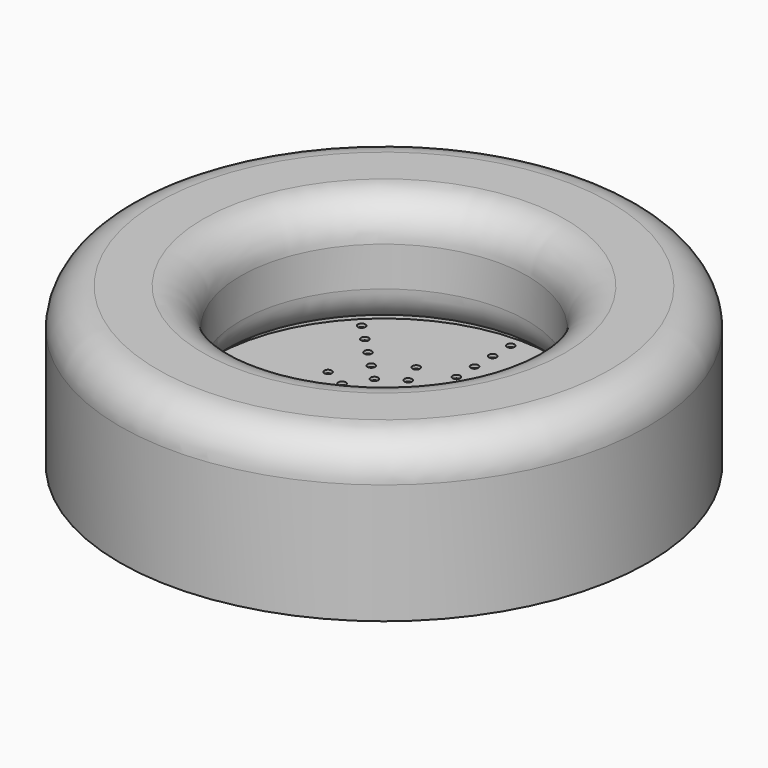
from build123d import *

# Parameters (mm, degrees)
F0_R      = 35
F0_R_2    = 20
F1_DEPTH  = 2
F2_R      = 35
F2_R_2    = 32
F3_DEPTH  = 3
F4_R      = 35
F5_DEPTH  = 0.4
F6_R      = 0.5
F7_DEPTH  = 1
F8_R      = 35
F8_R_2    = 22.5
F9_DEPTH  = 0.5
F10_R     = 35
F10_R_2   = 22.5
F10_R_3   = 19
F11_DEPTH = 15


# Not quite as in the source:
# - a fillet or chamfer that OpenCascade refuses, or shapes differently, is made with other operations: its cross-section is extruded or revolved along the edge and cut away or added


with BuildPart() as f1:
    # F0 (on Top) → F1 (new body)
    with BuildSketch(Plane.XY):
        Circle(F0_R)
        Circle(F0_R_2, mode=Mode.SUBTRACT)
    extrude(amount=F1_DEPTH)

    # F2 (on face) → F3 (join)
    with BuildSketch(Plane.XY.offset(2)):
        Circle(F2_R)
        Circle(F2_R_2, mode=Mode.SUBTRACT)
    extrude(amount=F3_DEPTH)

    # F4 (on face) → F5 (join)
    with BuildSketch(Plane.XY.offset(5)):
        Circle(F4_R)
    extrude(amount=F5_DEPTH)

    # F6 (on face) → F7 (cut)
    with BuildSketch(Plane.XY.offset(5.4)):
        Circle(F6_R)
        with Locations((3, 0)):
            Circle(F6_R)
        with Locations((6, 0)):
            Circle(F6_R)
        with Locations((9, 0)):
            Circle(F6_R)
        with Locations((12, 0)):
            Circle(F6_R)
        with Locations((15, 0)):
            Circle(F6_R)
        with Locations((18, 0)):
            Circle(F6_R)
        with Locations((21, 0)):
            Circle(F6_R)
        with Locations((2.1213203436, 2.1213203436)):
            Circle(F6_R)
        with Locations((4.2426406871, 4.2426406871)):
            Circle(F6_R)
        with Locations((6.3639610307, 6.3639610307)):
            Circle(F6_R)
        with Locations((8.4852813742, 8.4852813742)):
            Circle(F6_R)
        with Locations((10.6066017178, 10.6066017178)):
            Circle(F6_R)
        with Locations((12.7279220614, 12.7279220614)):
            Circle(F6_R)
        with Locations((14.8492424049, 14.8492424049)):
            Circle(F6_R)
        with Locations((0, 3)):
            Circle(F6_R)
        with Locations((0, 6)):
            Circle(F6_R)
        with Locations((0, 9)):
            Circle(F6_R)
        with Locations((0, 12)):
            Circle(F6_R)
        with Locations((0, 15)):
            Circle(F6_R)
        with Locations((0, 18)):
            Circle(F6_R)
        with Locations((0, 21)):
            Circle(F6_R)
        with Locations((-2.1213203436, 2.1213203436)):
            Circle(F6_R)
        with Locations((-4.2426406871, 4.2426406871)):
            Circle(F6_R)
        with Locations((-6.3639610307, 6.3639610307)):
            Circle(F6_R)
        with Locations((-8.4852813742, 8.4852813742)):
            Circle(F6_R)
        with Locations((-10.6066017178, 10.6066017178)):
            Circle(F6_R)
        with Locations((-12.7279220614, 12.7279220614)):
            Circle(F6_R)
        with Locations((-14.8492424049, 14.8492424049)):
            Circle(F6_R)
        with Locations((-3, 0)):
            Circle(F6_R)
        with Locations((-6, 0)):
            Circle(F6_R)
        with Locations((-9, 0)):
            Circle(F6_R)
        with Locations((-12, 0)):
            Circle(F6_R)
        with Locations((-15, 0)):
            Circle(F6_R)
        with Locations((-18, 0)):
            Circle(F6_R)
        with Locations((-21, 0)):
            Circle(F6_R)
        with Locations((-2.1213203436, -2.1213203436)):
            Circle(F6_R)
        with Locations((-4.2426406871, -4.2426406871)):
            Circle(F6_R)
        with Locations((-6.3639610307, -6.3639610307)):
            Circle(F6_R)
        with Locations((-8.4852813742, -8.4852813742)):
            Circle(F6_R)
        with Locations((-10.6066017178, -10.6066017178)):
            Circle(F6_R)
        with Locations((-12.7279220614, -12.7279220614)):
            Circle(F6_R)
        with Locations((-14.8492424049, -14.8492424049)):
            Circle(F6_R)
        with Locations((0, -3)):
            Circle(F6_R)
        with Locations((0, -6)):
            Circle(F6_R)
        with Locations((0, -9)):
            Circle(F6_R)
        with Locations((0, -12)):
            Circle(F6_R)
        with Locations((0, -15)):
            Circle(F6_R)
        with Locations((0, -18)):
            Circle(F6_R)
        with Locations((0, -21)):
            Circle(F6_R)
        with Locations((2.1213203436, -2.1213203436)):
            Circle(F6_R)
        with Locations((4.2426406871, -4.2426406871)):
            Circle(F6_R)
        with Locations((6.3639610307, -6.3639610307)):
            Circle(F6_R)
        with Locations((8.4852813742, -8.4852813742)):
            Circle(F6_R)
        with Locations((10.6066017178, -10.6066017178)):
            Circle(F6_R)
        with Locations((12.7279220614, -12.7279220614)):
            Circle(F6_R)
        with Locations((14.8492424049, -14.8492424049)):
            Circle(F6_R)
        with Locations((5.5432771951, 2.2961005942)):
            Circle(F6_R)
        with Locations((8.3149157926, 3.4441508913)):
            Circle(F6_R)
        with Locations((11.0865543901, 4.5922011884)):
            Circle(F6_R)
        with Locations((2.2961005942, 5.5432771951)):
            Circle(F6_R)
        with Locations((3.4441508913, 8.3149157926)):
            Circle(F6_R)
        with Locations((4.5922011884, 11.0865543901)):
            Circle(F6_R)
        with Locations((-2.2961005942, 5.5432771951)):
            Circle(F6_R)
        with Locations((-3.4441508913, 8.3149157926)):
            Circle(F6_R)
        with Locations((-4.5922011884, 11.0865543901)):
            Circle(F6_R)
        with Locations((-5.5432771951, 2.2961005942)):
            Circle(F6_R)
        with Locations((-8.3149157926, 3.4441508913)):
            Circle(F6_R)
        with Locations((-11.0865543901, 4.5922011884)):
            Circle(F6_R)
        with Locations((-5.5432771951, -2.2961005942)):
            Circle(F6_R)
        with Locations((-8.3149157926, -3.4441508913)):
            Circle(F6_R)
        with Locations((-11.0865543901, -4.5922011884)):
            Circle(F6_R)
        with Locations((-2.2961005942, -5.5432771951)):
            Circle(F6_R)
        with Locations((-3.4441508913, -8.3149157926)):
            Circle(F6_R)
        with Locations((-4.5922011884, -11.0865543901)):
            Circle(F6_R)
        with Locations((2.2961005942, -5.5432771951)):
            Circle(F6_R)
        with Locations((3.4441508913, -8.3149157926)):
            Circle(F6_R)
        with Locations((4.5922011884, -11.0865543901)):
            Circle(F6_R)
        with Locations((5.5432771951, -2.2961005942)):
            Circle(F6_R)
        with Locations((8.3149157926, -3.4441508913)):
            Circle(F6_R)
        with Locations((11.0865543901, -4.5922011884)):
            Circle(F6_R)
    extrude(amount=-F7_DEPTH, mode=Mode.SUBTRACT)

    # F8 (on face) → F9 (join)
    with BuildSketch(Plane.XY.offset(5.4)):
        Circle(F8_R)
        Circle(F8_R_2, mode=Mode.SUBTRACT)
    extrude(amount=F9_DEPTH)

    # F10 (on face) → F11 (join)
    with BuildSketch(Plane.XY.offset(5.9)):
        Circle(F10_R)
        Circle(F10_R_2, mode=Mode.SUBTRACT)
        Circle(F10_R_2)
        Circle(F10_R_3, mode=Mode.SUBTRACT)
    extrude(amount=F11_DEPTH)

    # F12: fillet of radius 5 on 4 edges, made by hand

    # F12_s1 → F12_t2 (revolve, cut)
    with BuildSketch(Plane.XZ):
        with BuildLine():
            ThreePointArc((24, 20.9), (20.4644660941, 19.4355339059), (19, 15.9))
            Line((19, 15.9), (19, 20.9))
            Line((19, 20.9), (24, 20.9))
        make_face()
    revolve(axis=Axis((0, 0, 20.9), (0, 0, 1)), mode=Mode.SUBTRACT)

    # F12_s3 → F12_t4 (revolve, cut)
    with BuildSketch(Plane.XZ):
        with BuildLine():
            ThreePointArc((35, 15.9), (33.5355339059, 19.4355339059), (30, 20.9))
            Line((30, 20.9), (35, 20.9))
            Line((35, 20.9), (35, 15.9))
        make_face()
    revolve(axis=Axis((0, 0, 20.9), (0, 0, 1)), mode=Mode.SUBTRACT)

    # F12_s5 → F12_t6 (revolve, cut)
    with BuildSketch(Plane.XZ):
        with BuildLine():
            ThreePointArc((19, 10.6696960071), (19.9688711259, 7.7116561155), (22.5, 5.9))
            Line((22.5, 5.9), (19, 5.9))
            Line((19, 5.9), (19, 10.6696960071))
        make_face()
    revolve(axis=Axis((0, 0, 5.9), (0, 0, 1)), mode=Mode.SUBTRACT)


solid = f1.part
